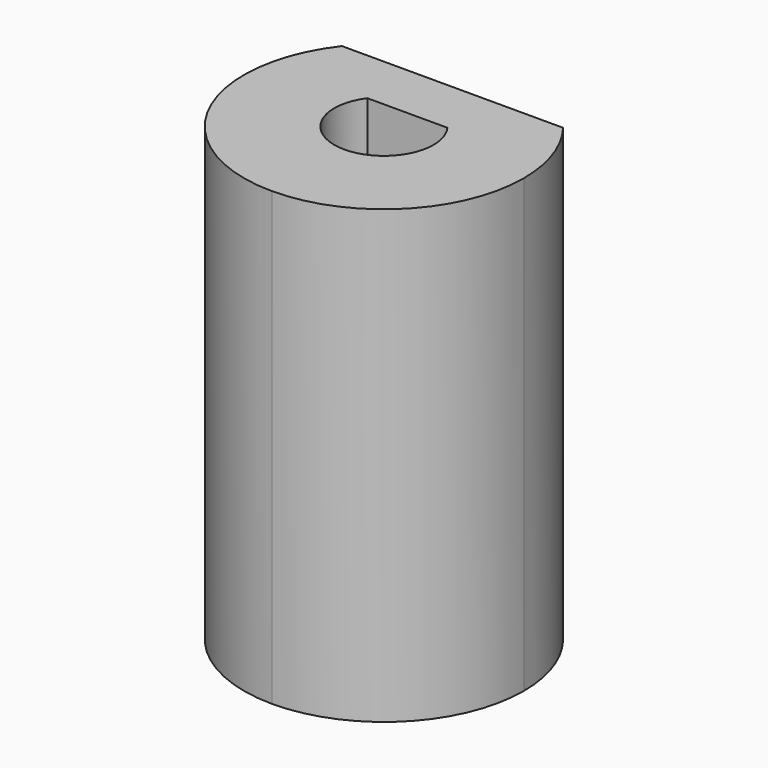
from build123d import *

# Parameters (mm, degrees)
F1_DEPTH = 10
F2_DEPTH = 4.7


with BuildPart() as f1:
    # F0 (on Top) → F1 (new body)
    with BuildSketch(Plane.XY):
        with BuildLine():
            ThreePointArc((0, -3.1), (2.1920310217, -2.1920310217), (3.1, 0))
            ThreePointArc((3.1, 0), (2.9328670446, 1.0041368924), (2.4494897428, 1.9))
            Line((2.4494897428, 1.9), (0, 1.9))
            Line((0, 1.9), (0, 1.1))
            ThreePointArc((0, 1.1), (0.4974937186, 0.9810708435), (0.8874119675, 0.65))
            ThreePointArc((0.8874119675, 0.65), (1.0455030283, 0.3419406643), (1.1, 0))
            ThreePointArc((1.1, 0), (0.7778174593, -0.7778174593), (0, -1.1))
            Line((0, -1.1), (0, -3.1))
        make_face()
        with BuildLine():
            ThreePointArc((-2.4494897428, 1.9), (-2.7838821814, -1.3638181697), (0, -3.1))
            Line((0, -3.1), (0, -1.1))
            ThreePointArc((0, -1.1), (-0.9810708435, -0.4974937186), (-0.8874119675, 0.65))
            ThreePointArc((-0.8874119675, 0.65), (-0.4974937186, 0.9810708435), (0, 1.1))
            Line((0, 1.1), (0, 1.9))
            Line((0, 1.9), (-2.4494897428, 1.9))
        make_face()
        with BuildLine():
            ThreePointArc((0.8874119675, 0.65), (0.4974937186, 0.9810708435), (0, 1.1))
            Line((0, 1.1), (0, 0.65))
            Line((0, 0.65), (0.8874119675, 0.65))
        make_face()
        with BuildLine():
            Line((0, 0.65), (0, 1.1))
            ThreePointArc((0, 1.1), (-0.4974937186, 0.9810708435), (-0.8874119675, 0.65))
            Line((-0.8874119675, 0.65), (0, 0.65))
        make_face()
    extrude(amount=F1_DEPTH)

    # F0 (on Top) → F2 (join)
    with BuildSketch(Plane.XY):
        with BuildLine():
            Line((0, 1.9), (2.4494897428, 1.9))
            ThreePointArc((2.4494897428, 1.9), (0, 3.1), (-2.4494897428, 1.9))
            Line((-2.4494897428, 1.9), (0, 1.9))
        make_face()
    extrude(amount=F2_DEPTH)


solid = f1.part
